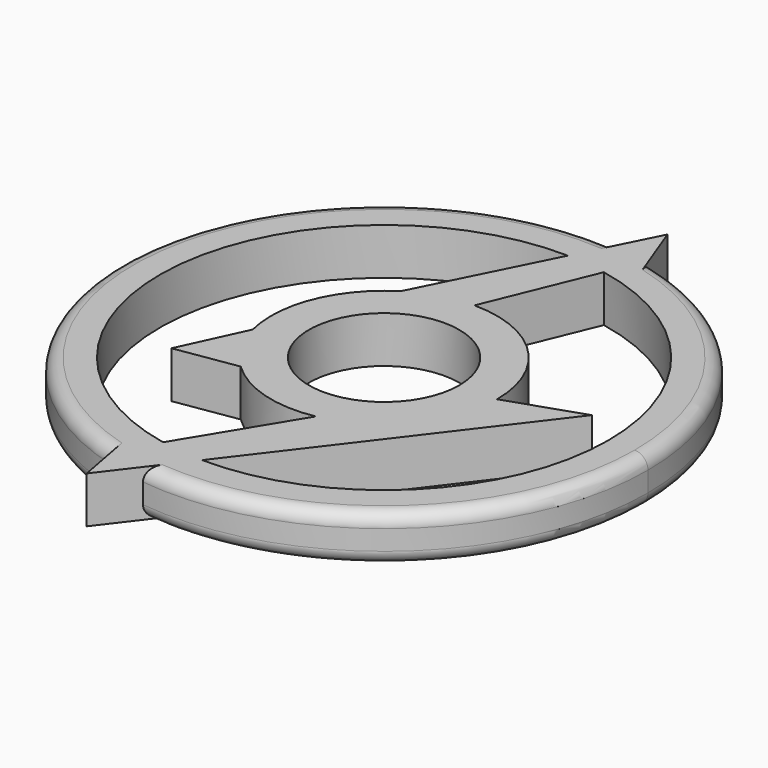
from build123d import *

# Parameters (mm, degrees)
F0_R     = 11.3
F1_DEPTH = 7
F2_R     = 2


# Not quite as in the source:
# - a feature names something its author has since deleted; it is built from what else it names


with BuildPart() as f1:
    # F0 (on Top) → F1 (new body)
    with BuildSketch(Plane.XY):
        with BuildLine():
            Line((8.8875694593, 38.6650469228), (6.5895106012, 33.0585853257))
            ThreePointArc((6.5895106012, 33.0585853257), (26.0616292761, 21.3795040442), (33.7089263208, 0))
            ThreePointArc((33.7089263208, 0), (23.6957200597, -23.9750821594), (-0.3950708864, -33.7066111126))
            Line((-0.3950708864, -33.7066111126), (-4.7252705017, -39.390945192))
            ThreePointArc((-4.7252705017, -39.390945192), (26.3297116519, -29.6769443973), (39.6733505572, 0))
            ThreePointArc((39.6733505572, 0), (31.0368684244, 24.7120930485), (8.8875694593, 38.6650469228))
        make_face()
        with BuildLine():
            ThreePointArc((0.6589035842, 33.7024859583), (3.6384789483, 33.5119856864), (6.5895106012, 33.0585853257))
            Line((6.5895106012, 33.0585853257), (8.8875694593, 38.6650469228))
            ThreePointArc((8.8875694593, 38.6650469228), (6.2429099817, 39.1790865053), (3.5694610238, 39.5124498409))
            Line((3.5694610238, 39.5124498409), (0.6589035842, 33.7024859583))
        make_face()
        with BuildLine():
            Line((-10.061211071, -38.3763830528), (-6.8087075048, -33.0141366056))
            ThreePointArc((-6.8087075048, -33.0141366056), (-33.4997306504, 3.7496346558), (0.6589035842, 33.7024859583))
            Line((0.6589035842, 33.7024859583), (3.5694610238, 39.5124498409))
            ThreePointArc((3.5694610238, 39.5124498409), (-39.0794482696, 6.8389668354), (-10.061211071, -38.3763830528))
        make_face()
        with BuildLine():
            ThreePointArc((-0.3950708864, -33.7066111126), (-3.6184922292, -33.5141496638), (-6.8087075048, -33.0141366056))
            Line((-6.8087075048, -33.0141366056), (-10.061211071, -38.3763830528))
            ThreePointArc((-10.061211071, -38.3763830528), (-7.4106236855, -38.9750869277), (-4.7252705017, -39.390945192))
            Line((-4.7252705017, -39.390945192), (-0.3950708864, -33.7066111126))
        make_face()
        with BuildLine():
            ThreePointArc((3.5694610238, 39.5124498409), (6.2429099817, 39.1790865053), (8.8875694593, 38.6650469228))
            Line((8.8875694593, 38.6650469228), (6.4280834783, 45.2187427282))
            Line((6.4280834783, 45.2187427282), (3.5694610238, 39.5124498409))
        make_face()
        with BuildLine():
            ThreePointArc((-4.7252705017, -39.390945192), (-7.4106236855, -38.9750869277), (-10.061211071, -38.3763830528))
            Line((-10.061211071, -38.3763830528), (-8.8514386924, -44.8074434017))
            Line((-8.8514386924, -44.8074434017), (-4.7252705017, -39.390945192))
        make_face()
        with BuildLine():
            ThreePointArc((-9.0146919562, 14.392356585), (-4.6897069772, 16.3221091653), (0, 16.9824791811))
            Line((0, 16.9824791811), (6.5895106012, 33.0585853257))
            ThreePointArc((6.5895106012, 33.0585853257), (3.6384789483, 33.5119856864), (0.6589035842, 33.7024859583))
            Line((0.6589035842, 33.7024859583), (-9.0146919562, 14.392356585))
        make_face()
        with BuildLine():
            ThreePointArc((3.0870048037, -16.6995509065), (13.054301857, -10.8623110875), (16.9824791811, 0))
            ThreePointArc((16.9824791811, 0), (12.0084261903, 12.0084261903), (0, 16.9824791811))
            ThreePointArc((0, 16.9824791811), (-4.6897069772, 16.3221091653), (-9.0146919562, 14.392356585))
            ThreePointArc((-9.0146919562, 14.392356585), (-15.7401759471, 6.37584977), (-16.4896996402, -4.0613304363))
            ThreePointArc((-16.4896996402, -4.0613304363), (-14.690740637, -8.5197851306), (-11.7143980752, -12.2954250382))
            ThreePointArc((-11.7143980752, -12.2954250382), (-4.8432488922, -16.2772091989), (3.0870048037, -16.6995509065))
        make_face()
        Circle(F0_R, mode=Mode.SUBTRACT)
        with BuildLine():
            Line((-20.9624820809, -13.7546608704), (-11.7143980752, -12.2954250382))
            ThreePointArc((-11.7143980752, -12.2954250382), (-14.690740637, -8.5197851306), (-16.4896996402, -4.0613304363))
            Line((-16.4896996402, -4.0613304363), (-20.9624820809, -13.7546608704))
        make_face()
        with BuildLine():
            Line((28.1798244973, 3.8041888679), (16.9824791811, 0))
            ThreePointArc((16.9824791811, 0), (13.054301857, -10.8623110875), (3.0870048037, -16.6995509065))
            Line((3.0870048037, -16.6995509065), (-6.8087075048, -33.0141366056))
            ThreePointArc((-6.8087075048, -33.0141366056), (-3.6184922292, -33.5141496638), (-0.3950708864, -33.7066111126))
            Line((-0.3950708864, -33.7066111126), (28.1798244973, 3.8041888679))
        make_face()
    extrude(amount=F1_DEPTH)

    # F2
    f2_edges = [f1.edges().sort_by_distance(p)[0] for p in [
        (39.083445, -6.81609, 7),
        (39.083445, -6.81609, 0),
        (-39.079448, 6.838967, 0),
        (-39.079448, 6.838967, 7),
    ]]
    fillet(f2_edges, radius=F2_R)


solid = f1.part
